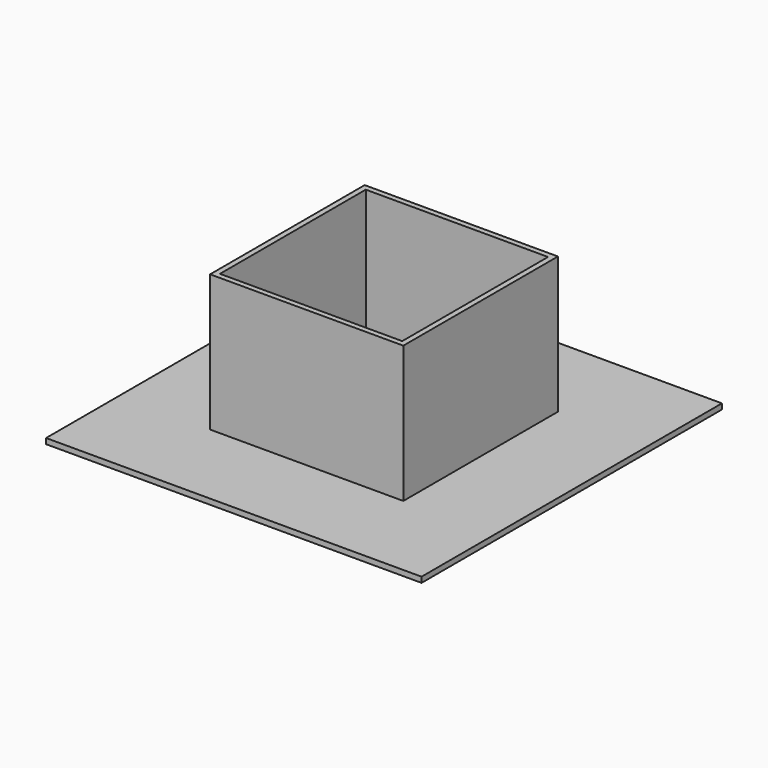
from build123d import *

# Parameters (mm, degrees)
F0_W     = 206
F0_H     = 206
F0_W_2   = 100
F0_H_2   = 100
F1_DEPTH = 3
F2_W     = 106
F2_H     = 106
F2_W_2   = 100
F2_H_2   = 100
F3_DEPTH = 75


# Not quite as in the source:
# - a feature names something its author has since deleted; it is built from what else it names


with BuildPart() as f1:
    # F0 (on Top) → F1 (new body)
    with BuildSketch(Plane.XY):
        Rectangle(F0_W, F0_H)
        Rectangle(F0_W_2, F0_H_2, mode=Mode.SUBTRACT)
    extrude(amount=F1_DEPTH)

    # F2 (on face) → F3 (join)
    with BuildSketch(Plane.XY.offset(3)):
        Rectangle(F2_W, F2_H)
        Rectangle(F2_W_2, F2_H_2, mode=Mode.SUBTRACT)
    extrude(amount=F3_DEPTH)


solid = f1.part
